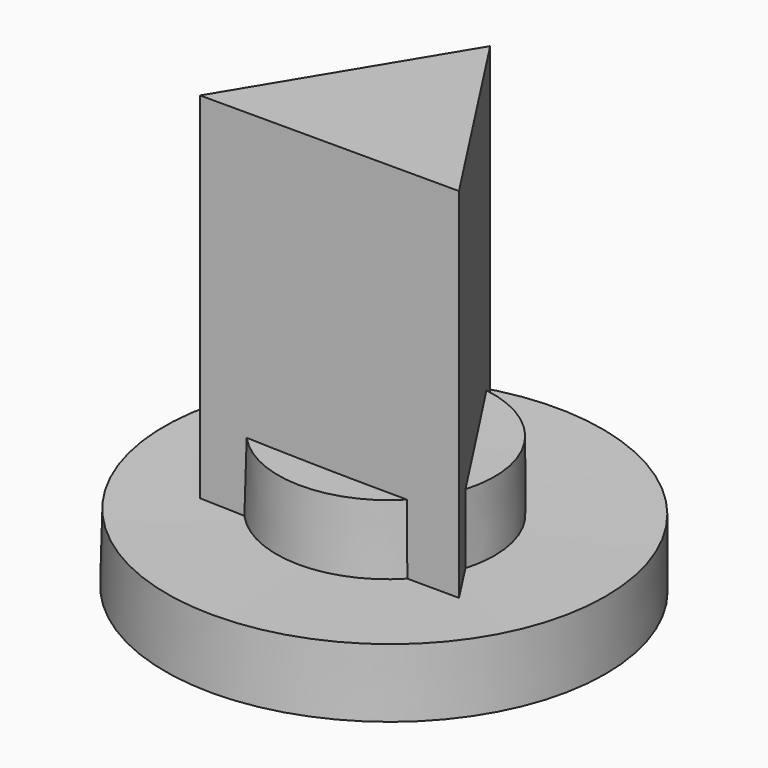
from build123d import *

# Parameters (mm, degrees)
F3_DEPTH = 74.9529767781


with BuildPart() as f1:
    # F0 (on Front) → F1 (revolve)
    with BuildSketch(Plane.XZ):
        Polygon((0.4052141029, 14.5266056061), (0.2008356291, 0), (23.175150156, 0), (23.175150156, 14.5266056061), (11.587575078, 14.5266056061), align=None)
        Polygon((0.2008356291, 0), (0, -14.2747908831), (46.350300312, -14.2747908831), (46.350300312, 0), (23.175150156, 0), align=None)
        Polygon((0.9806752205, 55.4286465049), (0.4052141029, 14.5266056061), (11.587575078, 14.5266056061), (11.9791924953, 55.4286465049), align=None)
    revolve(axis=Axis((0.4903376102, 0, 20.5769278109), (-0.0140678597, 0, -0.9999010428)))

    # F2 (on Top) → F3 (join)
    with BuildSketch(Plane.XY):
        Polygon((-26.0949339381, -15.407031402), (28.0455284658, -15.407031402), (0, 27.8120934963), align=None)
    extrude(amount=F3_DEPTH)


solid = f1.part
